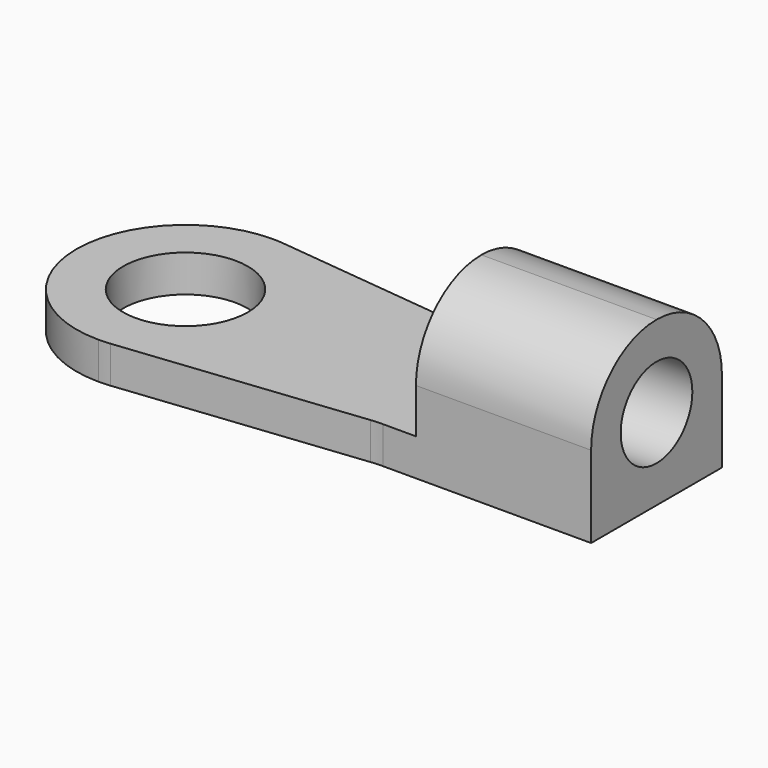
from build123d import *

# Parameters (mm, degrees)
F0_R     = 1.6
F1_DEPTH = 0.95
F2_W     = 4.5
F2_H     = 4.2
F3_DEPTH = 3.25
F4_R     = 2.09999
F5_R     = 1.15
F6_DEPTH = 25


# Not quite as in the source:
# - a fillet or chamfer is up to 0.001 mm smaller than in the source, because OpenCascade refuses the exact size


with BuildPart() as f1:
    # F0 (on Top) → F1 (new body)
    with BuildSketch(Plane.XY):
        with BuildLine():
            Line((9.5515289224, 0.7), (14.9, 0.7))
            Line((14.9, 0.7), (14.9, 4.9))
            Line((14.9, 4.9), (9.5515289224, 4.9))
            ThreePointArc((9.5515289224, 4.9), (9.4002214052, 4.9040911969), (9.2493560516, 4.916352832))
            Line((9.2493560516, 4.916352832), (3.1021728708, 5.583647168))
            ThreePointArc((3.1021728708, 5.583647168), (2.9513075171, 5.5959088031), (2.8, 5.6))
            ThreePointArc((2.8, 5.6), (0.8201010127, 4.7798989873), (0, 2.8))
            ThreePointArc((0, 2.8), (0.8201010127, 0.8201010127), (2.8, 0))
            ThreePointArc((2.8, 0), (2.9513075171, 0.0040911969), (3.1021728708, 0.016352832))
            Line((3.1021728708, 0.016352832), (9.2493560516, 0.683647168))
            ThreePointArc((9.2493560516, 0.683647168), (9.4002214052, 0.6959088031), (9.5515289224, 0.7))
        make_face()
        with Locations((2.8, 2.8)):
            Circle(F0_R, mode=Mode.SUBTRACT)
    extrude(amount=F1_DEPTH)

    # F2 (on face) → F3 (join)
    with BuildSketch(Plane.XY.offset(0.95)):
        with Locations((12.65, 2.8)):
            Rectangle(F2_W, F2_H)
    extrude(amount=F3_DEPTH)

    # F4 (radius 2.1 in the source; OpenCascade refuses exactly that, so slightly less here)
    f4_edges = [f1.edges().sort_by_distance(p)[0] for p in [
        (12.65, 0.7, 4.2),
        (12.65, 4.9, 4.2),
    ]]
    fillet(f4_edges, radius=F4_R)

    # F5 (on face) → F6 (cut)
    with BuildSketch(Plane.YZ.offset(14.9)):
        with Locations((2.8, 2.1)):
            Circle(F5_R)
    extrude(amount=-F6_DEPTH, mode=Mode.SUBTRACT)


solid = f1.part
